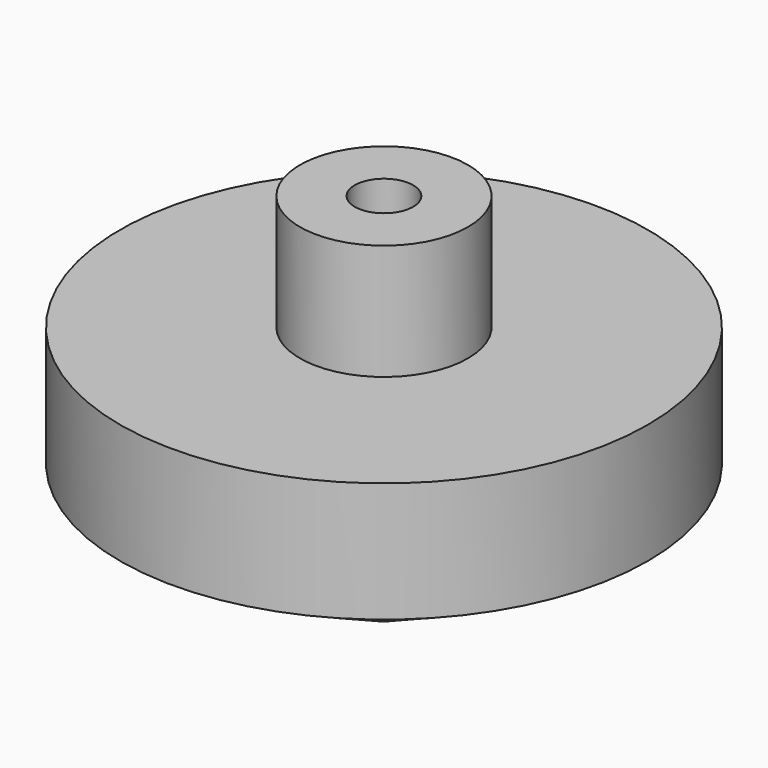
from build123d import *

# Parameters (mm, degrees)
F3_D     = 9.906
F3_DEPTH = 9.525
F3_TIP   = 2.976062646


with BuildPart() as f1:
    # F0 (on Front) → F1 (revolve)
    with BuildSketch(Plane.XZ):
        Polygon((0, 63.5), (0, 0), (44.7203114587, 23.5954719484), (44.7203114587, 43.9154719484), (14.2403114587, 43.9154719484), (14.2403114587, 63.5), align=None)
    revolve(axis=Axis((0, 0, 31.75), (0, 0, -1)))

    # F3
    with Locations(Plane.XY.offset(63.5)):
        with Locations((0, 0)):
            Hole(F3_D / 2, depth=F3_DEPTH)
            with Locations((0, 0, -(F3_DEPTH + F3_TIP / 2))):  # 118° drill point
                Cone(0, F3_D / 2, F3_TIP, mode=Mode.SUBTRACT)


solid = f1.part
